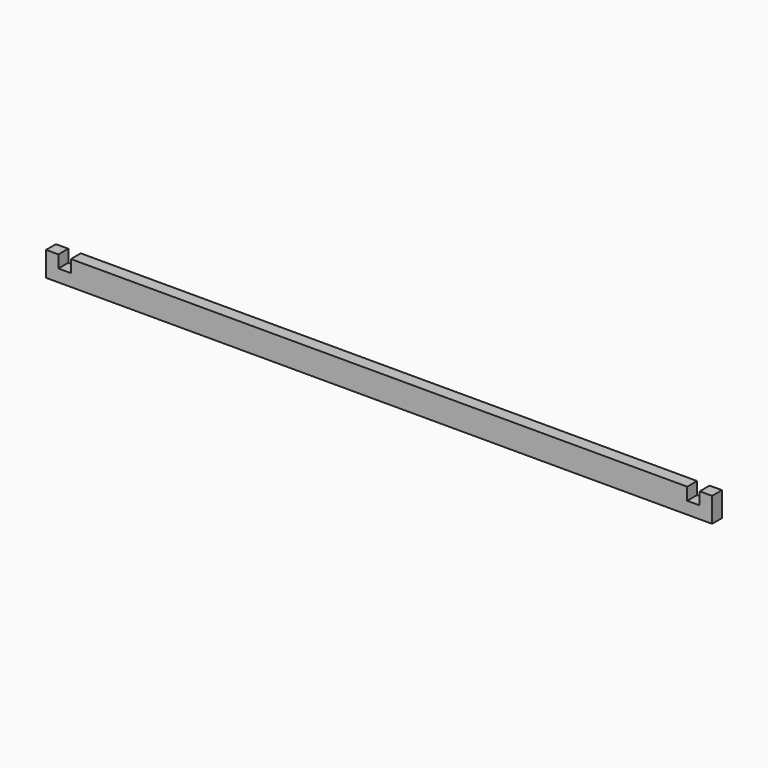
from build123d import *

# Parameters (mm, degrees)
F1_DEPTH = 3


# Not quite as in the source:
# - a feature names something its author has since deleted; it is built from what else it names


with BuildPart() as f1:
    # F0 (on Front) → F1 (new body)
    with BuildSketch(Plane.XZ):
        Polygon((-81.04, 6), (-81.04, 0), (81.04, 0), (81.04, 6), (78.04, 6), (78.04, 2.98), (75, 2.98), (75, 6), (-75, 6), (-75, 2.98), (-78.04, 2.98), (-78.04, 6), align=None)
    extrude(amount=F1_DEPTH)


solid = f1.part
